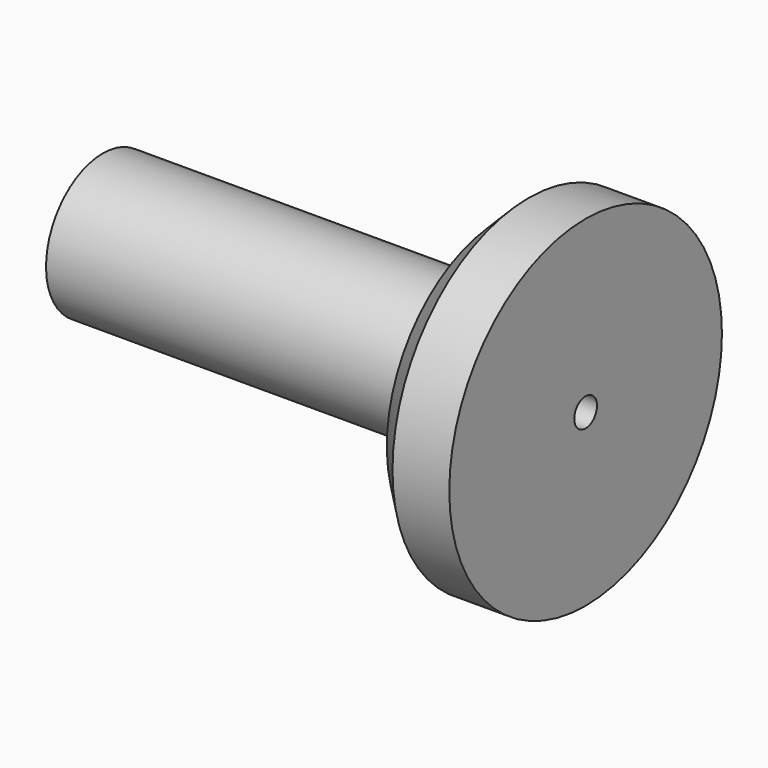
from build123d import *

# Parameters (mm, degrees)
F3_D     = 8.8
F3_DEPTH = 28.75
F3_TIP   = 2.6437867237
F5_D     = 5


# Not quite as in the source:
# - a feature names something its author has since deleted; it is built from what else it names


with BuildPart() as f1:
    # F0 (on Front) → F1 (revolve)
    with BuildSketch(Plane.XZ):
        Polygon((23.7903209624, 12.5), (-46.2096790376, 12.5), (-46.2096790376, 0), (38.7903209624, 0), (38.7903209624, 30), (28.7903209624, 30), (23.7903209624, 25), align=None)
    revolve(axis=Axis((-0.8820928633, 0, 0), (1, 0, 0)))

    # F3
    with Locations(Plane(origin=(-46.2096790376, 0, 0), x_dir=(0, -1, 0), z_dir=(-1, 0, 0))):
        with Locations((0, 0)):
            Hole(F3_D / 2, depth=F3_DEPTH)
            with Locations((0, 0, -(F3_DEPTH + F3_TIP / 2))):  # 118° drill point
                Cone(0, F3_D / 2, F3_TIP, mode=Mode.SUBTRACT)

    # F5 (through all)
    with Locations(Plane.YZ.offset(38.7903209624)):
        with Locations((0, 0)):
            Hole(F5_D / 2)


solid = f1.part
